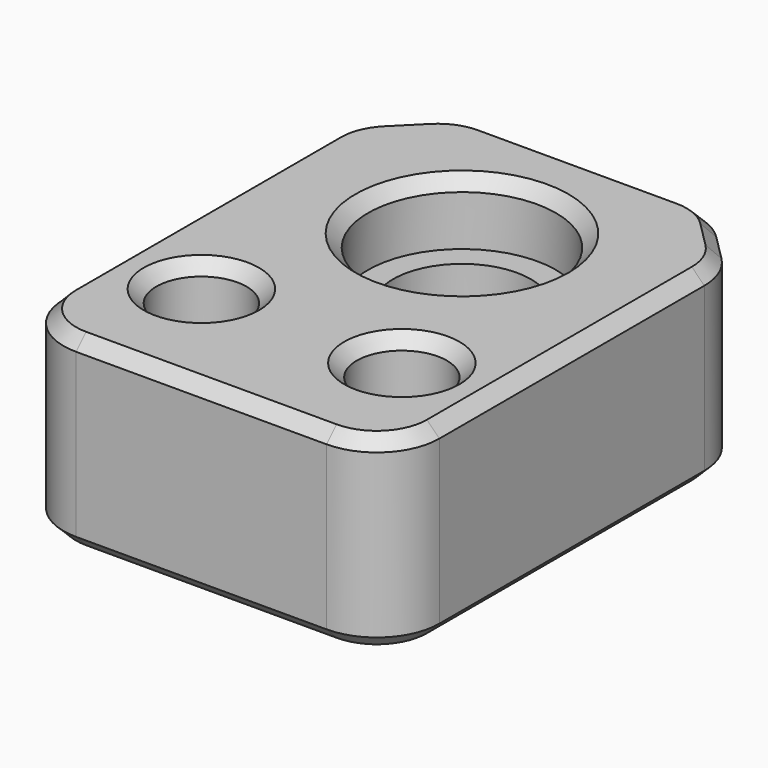
from build123d import *

# Parameters (mm, degrees)
F0_W     = 30
F0_H     = 38.5
F0_R     = 3.6
F0_R_2   = 7.5
F1_DEPTH = 15
F0_R_3   = 2.15
F2_DEPTH = 5
F3_START = 5
F0_R_4   = 5.5
F3_DEPTH = 5
F4_SIZE  = 1.99999
F5_SIZE  = 5
F6_R     = 5
F7_R     = 5
F8_SIZE  = 1


# Not quite as in the source:
# - a fillet or chamfer is up to 0.001 mm smaller than in the source, because OpenCascade refuses the exact size


with BuildPart() as f1:
    # F0 (on Top) → F1 (new body)
    with BuildSketch(Plane.XY):
        Rectangle(F0_W, F0_H)
        with Locations((-8, -9.25)):
            Circle(F0_R, mode=Mode.SUBTRACT)
        with Locations((8, -9.25)):
            Circle(F0_R, mode=Mode.SUBTRACT)
        with Locations((0, 6.75)):
            Circle(F0_R_2, mode=Mode.SUBTRACT)
    extrude(amount=F1_DEPTH)

    # F0 (on Top) → F2 (join)
    with BuildSketch(Plane.XY):
        with Locations((-8, -9.25)):
            Circle(F0_R)
        with Locations((-8, -9.25)):
            Circle(F0_R_3, mode=Mode.SUBTRACT)
        with Locations((8, -9.25)):
            Circle(F0_R)
        with Locations((8, -9.25)):
            Circle(F0_R_3, mode=Mode.SUBTRACT)
    extrude(amount=F2_DEPTH)

    # F0 (on Top) → F3 (join)
    with BuildSketch(Plane.XY.offset(F3_START)):
        with Locations((0, 6.75)):
            Circle(F0_R_2)
        with Locations((0, 6.75)):
            Circle(F0_R_4, mode=Mode.SUBTRACT)
    extrude(amount=F3_DEPTH)

    # F4 (size 2 in the source; OpenCascade refuses exactly that, so slightly less here)
    f4_edges = [f1.edges().sort_by_distance(p)[0] for p in [
        (-5.5, 6.75, 5),
    ]]
    chamfer(f4_edges, length=F4_SIZE)

    # F5
    f5_edges = [f1.edges().sort_by_distance(p)[0] for p in [
        (15, 19.25, 7.5),
        (-15, 19.25, 7.5),
    ]]
    chamfer(f5_edges, length=F5_SIZE)

    # F6
    f6_edges = [f1.edges().sort_by_distance(p)[0] for p in [
        (15, -19.25, 7.5),
        (-15, -19.25, 7.5),
    ]]
    fillet(f6_edges, radius=F6_R)

    # F7
    f7_edges = [f1.edges().sort_by_distance(p)[0] for p in [
        (15, 14.25, 7.5),
        (10, 19.25, 7.5),
        (-10, 19.25, 7.5),
        (-15, 14.25, 7.5),
    ]]
    fillet(f7_edges, radius=F7_R)

    # F8
    f8_edges = [f1.edges().sort_by_distance(p)[0] for p in [
        (15, -1.035534, 15),
        (14.619398, 14.092349, 15),
        (13.535534, -17.785534, 15),
        (12.5, 16.75, 15),
        (0, -19.25, 15),
        (9.842349, 18.869398, 15),
        (-13.535534, -17.785534, 15),
        (0, 19.25, 15),
        (-15, -1.035534, 15),
        (-9.842349, 18.869398, 15),
        (-14.619398, 14.092349, 15),
        (-12.5, 16.75, 15),
        (-11.6, -9.25, 15),
        (4.4, -9.25, 15),
        (-7.5, 6.75, 15),
        (15, -1.035534, 0),
        (14.619398, 14.092349, 0),
        (13.535534, -17.785534, 0),
        (12.5, 16.75, 0),
        (0, -19.25, 0),
        (9.842349, 18.869398, 0),
        (-13.535534, -17.785534, 0),
        (0, 19.25, 0),
        (-15, -1.035534, 0),
        (-9.842349, 18.869398, 0),
        (-14.619398, 14.092349, 0),
        (-12.5, 16.75, 0),
        (-7.5, 6.75, 0),
        (-10.15, -9.25, 0),
        (5.85, -9.25, 0),
    ]]
    chamfer(f8_edges, length=F8_SIZE)


solid = f1.part
